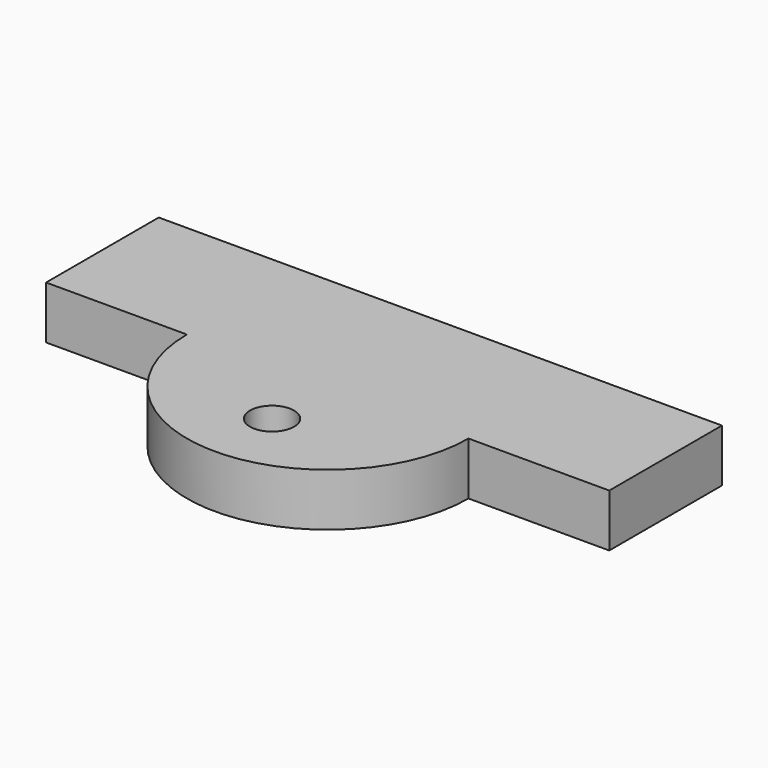
from build123d import *

# Parameters (mm, degrees)
F0_R     = 7.9375
F1_DEPTH = 19.05


# Not quite as in the source:
# - a feature of the source that left no trace in its solid (it failed there, or was rolled back) is left out


with BuildPart() as f1:
    # F0 (on Top) → F1 (new body)
    with BuildSketch(Plane.XY):
        with BuildLine():
            ThreePointArc((-253.1241280528, -50.8), (-238.245152537, -14.8789755157), (-202.3241280528, 0))
            Line((-202.3241280528, 0), (-303.9241280528, 0))
            Line((-303.9241280528, 0), (-303.9241280528, -50.8))
            Line((-303.9241280528, -50.8), (-253.1241280528, -50.8))
        make_face()
        with BuildLine():
            ThreePointArc((-151.5241280528, -50.8), (-166.4031035685, -14.8789755157), (-202.3241280528, 0))
            ThreePointArc((-202.3241280528, 0), (-238.245152537, -14.8789755157), (-253.1241280528, -50.8))
            Line((-253.1241280528, -50.8), (-151.5241280528, -50.8))
        make_face()
        with BuildLine():
            Line((-100.7241280528, -50.8), (-100.7241280528, 0))
            Line((-100.7241280528, 0), (-202.3241280528, 0))
            ThreePointArc((-202.3241280528, 0), (-166.4031035685, -14.8789755157), (-151.5241280528, -50.8))
            Line((-151.5241280528, -50.8), (-100.7241280528, -50.8))
        make_face()
        with BuildLine():
            ThreePointArc((-253.1241280528, -50.8), (-202.3241280528, -101.6), (-151.5241280528, -50.8))
            Line((-151.5241280528, -50.8), (-253.1241280528, -50.8))
        make_face()
        with Locations((-202.3241280528, -75.8825)):
            Circle(F0_R, mode=Mode.SUBTRACT)
    extrude(amount=F1_DEPTH)


solid = f1.part
